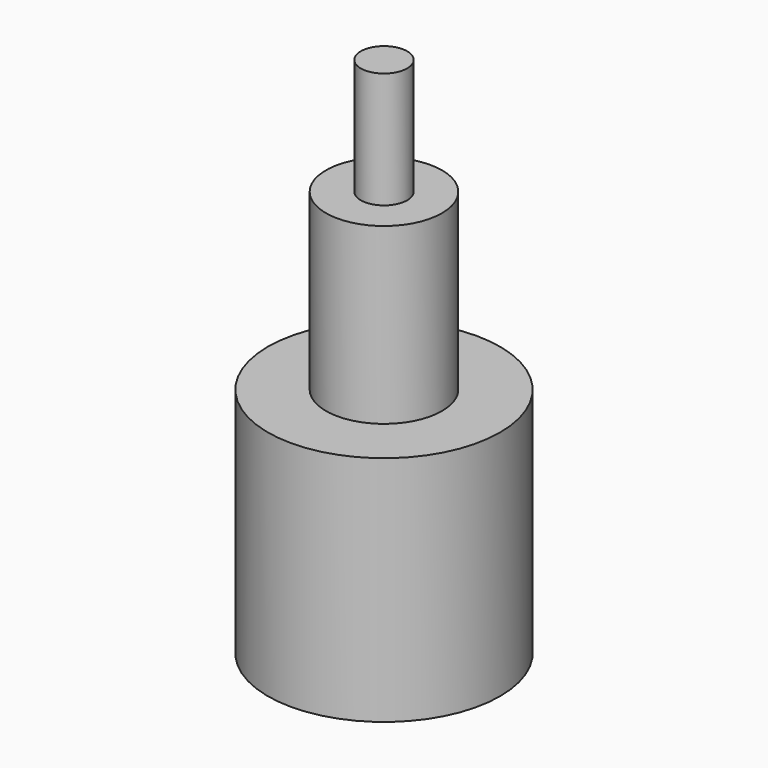
from build123d import *

# Parameters (mm, degrees)
F0_R      = 25
F2_DEPTH  = 50
F3_R      = 12.5
F4_DEPTH  = 37.5
F10_D     = 10
F10_DEPTH = 25
F10_TIP   = 3.0043030951
F11_R     = 5
F12_DEPTH = 25


# Not quite as in the source:
# - a feature of the source that left no trace in its solid (it failed there, or was rolled back) is left out


with BuildPart() as f2:
    # F0 (on Top) → F2 (new body)
    with BuildSketch(Plane.XY):
        Circle(F0_R)
    extrude(amount=F2_DEPTH)

    # F3 (on face) → F4 (join)
    with BuildSketch(Plane.XY.offset(50)):
        Circle(F3_R)
    extrude(amount=F4_DEPTH)

    # F10
    with Locations(Plane(origin=(0, 0, 0), x_dir=(1, 0, 0), z_dir=(0, 0, -1))):
        with Locations((0, 0)):
            Hole(F10_D / 2, depth=F10_DEPTH)
            with Locations((0, 0, -(F10_DEPTH + F10_TIP / 2))):  # 118° drill point
                Cone(0, F10_D / 2, F10_TIP, mode=Mode.SUBTRACT)

    # F11 (on face) → F12 (join)
    with BuildSketch(Plane.XY.offset(87.5)):
        Circle(F11_R)
    extrude(amount=F12_DEPTH)


solid = f2.part
